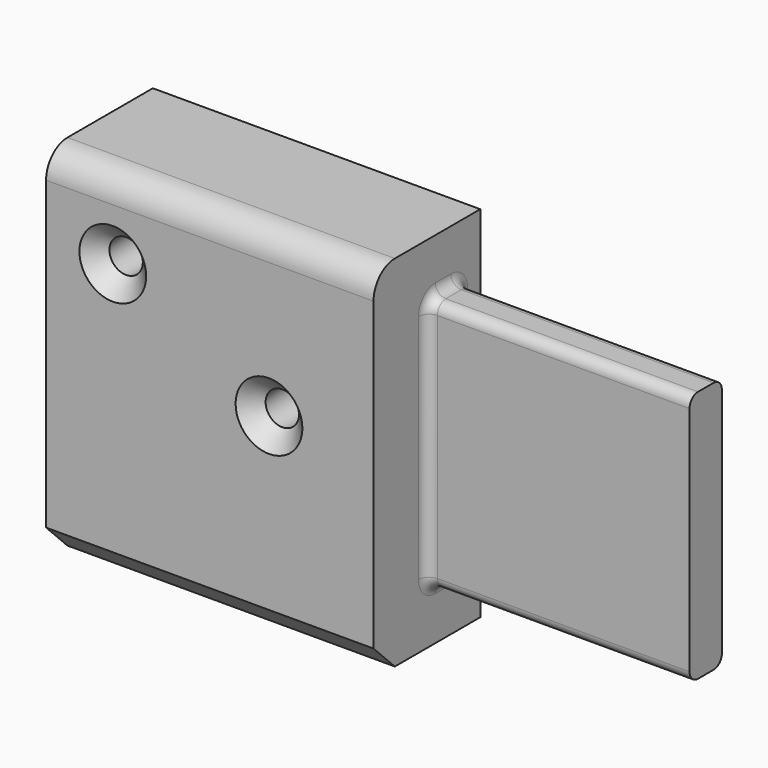
from build123d import *

# Parameters (mm, degrees)
F0_W           = 62.330626417
F0_H           = 68.3823013678
F1_DEPTH       = 12.7
F3_D           = 6.35
F3_CSINK_D     = 12.7
F3_CSINK_ANGLE = 90
F4_R           = 5.08
F5_SIZE        = 5.08
F6_W           = 42.330626417
F6_H           = 20
F7_DEPTH       = 20
F8_R           = 9.99999
F9_W           = 7.7
F9_H           = 48.0895394087
F10_DEPTH      = 50
F11_F1_R       = 2
F11_F2_R       = 2


# Not quite as in the source:
# - a fillet or chamfer is up to 0.001 mm smaller than in the source, because OpenCascade refuses the exact size


with BuildPart() as f1:
    # F0 (on Front) → F1 (new body, symmetric)
    with BuildSketch(Plane.XZ):
        with Locations((-36.5127732512, 23.8983887248)):
            Rectangle(F0_W, F0_H)
    extrude(amount=F1_DEPTH, both=True)

    # F3 (through all)
    with Locations(Plane.XZ.offset(12.7)):
        with Locations((-54.9780864596, 43.1276711741), (-25.2489887894, 27.2838656685)):
            CounterSinkHole(F3_D / 2, F3_CSINK_D / 2, counter_sink_angle=F3_CSINK_ANGLE)

    # F4
    f4_edges = [f1.edges().sort_by_distance(p)[0] for p in [
        (-36.512773, -12.7, 58.089539),
    ]]
    fillet(f4_edges, radius=F4_R)

    # F5
    f5_edges = [f1.edges().sort_by_distance(p)[0] for p in [
        (-36.512773, -12.7, -10.292762),
    ]]
    chamfer(f5_edges, length=F5_SIZE)

    # F6 (on face) → F7 (join)
    with BuildSketch(Plane(origin=(0, 12.7, 0), x_dir=(-1, 0, 0), z_dir=(0, 1, 0))):
        with Locations((36.5127732512, 9.7072380409)):
            Rectangle(F6_W, F6_H)
    extrude(amount=F7_DEPTH)

    # F8 (radius 10 in the source; OpenCascade refuses exactly that, so slightly less here)
    f8_edges = [f1.edges().sort_by_distance(p)[0] for p in [
        (-15.34746, 22.7, 19.707238),
        (-15.34746, 22.7, -0.292762),
        (-57.678086, 22.7, 19.707238),
        (-57.678086, 22.7, -0.292762),
    ]]
    fillet(f8_edges, radius=F8_R)

    # F9 (on face) → F10 (join)
    with BuildSketch(Plane.YZ.offset(-5.3474600427)):
        with Locations((3.85, 24.0447697043)):
            Rectangle(F9_W, F9_H)
    extrude(amount=F10_DEPTH)

    # F11: fillet of radius 2 on 6 edges, made by hand

    # F11_f1
    f11_f1_edges = [f1.edges().sort_by_distance(p)[0] for p in [
        (19.6525399573, 7.7, 48.0895394087),
        (19.6525399573, 0, 48.0895394087),
        (19.6525399573, 7.7, 0),
        (19.6525399573, 0, 0),
    ]]
    fillet(f11_f1_edges, radius=F11_F1_R)

    # F11_f2
    f11_f2_edges = [f1.edges().sort_by_distance(p)[0] for p in [
        (-5.3474600427, 0, 24.0447697043),
        (-5.3474600427, 7.7, 24.0447697043),
        (-5.3474600427, 7.1142135624, 0.5857864376),
        (-5.3474600427, 7.1142135624, 47.5037529711),
        (-5.3474600427, 0.5857864376, 47.5037529711),
        (-5.3474600427, 0.5857864376, 0.5857864376),
    ]]
    fillet(f11_f2_edges, radius=F11_F2_R)


solid = f1.part
